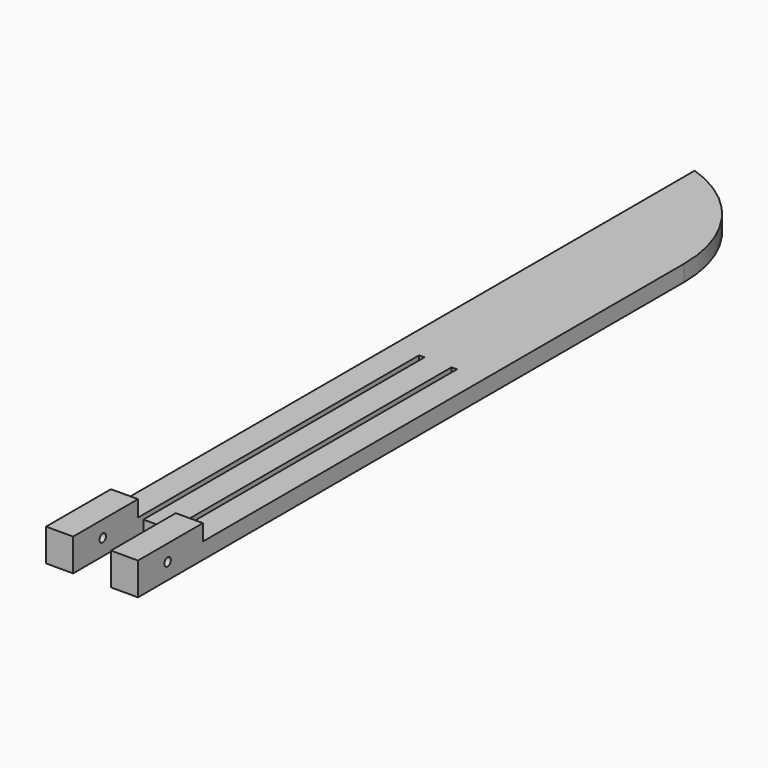
from build123d import *

# Parameters (mm, degrees)
F1_DEPTH    = 6
F2_W        = 10
F2_H        = 30
F3_DEPTH    = 6
F4_R        = 1.5
F5_DEPTH    = 34.001
F6_T1_DEPTH = 242.8543856465


# Not quite as in the source:
# - a fillet or chamfer that OpenCascade refuses, or shapes differently, is made with other operations: its cross-section is extruded or revolved along the edge and cut away or added


with BuildPart() as f1:
    # F0 (on Top) → F1 (new body)
    with BuildSketch(Plane.XY):
        Polygon((7, -150), (17, -150), (17, 150), (-17, 150), (-17, -150), (-7, -150), (-7, 10), (-5, 10), (-5, -120), (5, -120), (5, 10), (7, 10), align=None)
    extrude(amount=F1_DEPTH)

    # F2 (on face) → F3 (join)
    with BuildSketch(Plane.XY.offset(6)):
        with Locations((-12, -135)):
            Rectangle(F2_W, F2_H)
        with Locations((12, -135)):
            Rectangle(F2_W, F2_H)
    extrude(amount=F3_DEPTH)

    # F4 (on face) → F5 (cut, through all)
    with BuildSketch(Plane(origin=(-17, 0, 0), x_dir=(0, -1, 0), z_dir=(-1, 0, 0))):
        with Locations((136.3040655851, 6)):
            Circle(F4_R)
    extrude(amount=-F5_DEPTH, mode=Mode.SUBTRACT)

    # F6: fillet of radius 50 on 1 edges, made by hand

    # F6_s2 → F6_t1 (cut)
    with BuildSketch(Plane.XY.offset(-118.4271928233)):
        with BuildLine():
            ThreePointArc((17, 102.6291228707), (7.6201920232, 131.7838823449), (-17, 150))
            Line((-17, 150), (17, 150))
            Line((17, 150), (17, 102.6291228707))
        make_face()
    extrude(amount=F6_T1_DEPTH, mode=Mode.SUBTRACT)


solid = f1.part
